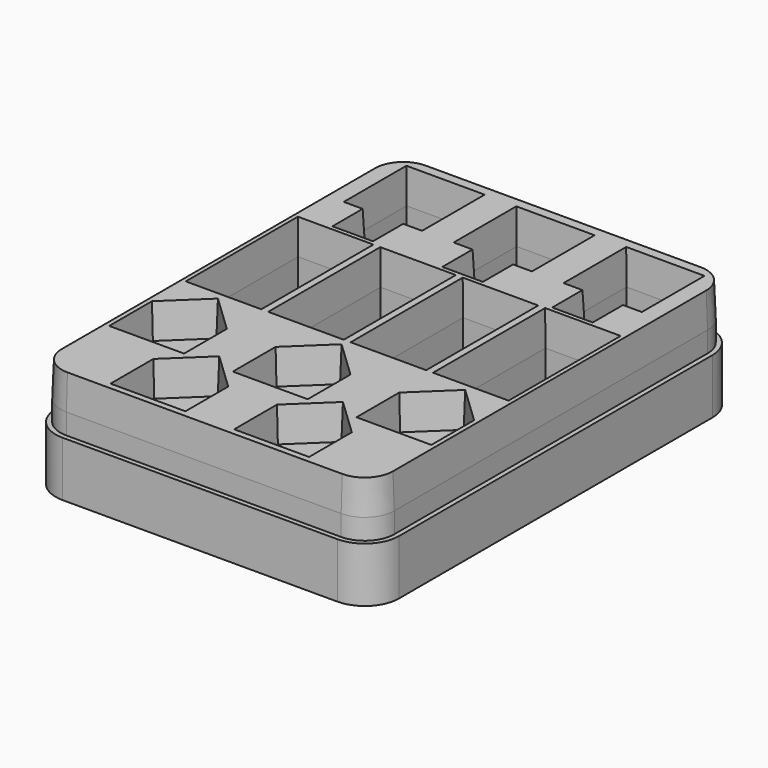
from build123d import *

# Parameters (mm, degrees)
F1_DEPTH = 1
F0_W     = 10.6
F0_H     = 20
F2_DEPTH = 7
F3_DEPTH = 11
F4_DEPTH = 16
F5_DEPTH = 8
F6_SIZE2 = 4.99999
F6_SIZE  = 0.19999


# Not quite as in the source:
# - a fillet or chamfer is up to 0.001 mm smaller than in the source, because OpenCascade refuses the exact size


with BuildPart() as f1:
    # F0 (on Top) → F1 (new body)
    with BuildSketch(Plane.XY):
        Polygon((-18.75, 14.5), (-13.25, 14.5), (-13.25, 20), (-10.5, 20), (-10.5, 31), (-21.5, 31), (-21.5, 20), (-18.75, 20), align=None)
    extrude(amount=F1_DEPTH)



with BuildPart() as f1b:
    # F0 (on Top) → F1, piece 2 (new body)
    with BuildSketch(Plane.XY):
        Polygon((5.5, 31), (-5.5, 31), (-5.5, 20), (-2.75, 20), (-2.75, 14.5), (2.75, 14.5), (2.75, 20), (5.5, 20), align=None)
    extrude(amount=F1_DEPTH)


with BuildPart() as f1c:
    # F0 (on Top) → F1, piece 3 (new body)
    with BuildSketch(Plane.XY):
        Polygon((21.5, 31), (10.5, 31), (10.5, 20), (13.25, 20), (13.25, 14.5), (18.75, 14.5), (18.75, 20), (21.5, 20), align=None)
    extrude(amount=F1_DEPTH)


with BuildPart() as f2:
    # F0 (on Top) → F2 (new body)
    with BuildSketch(Plane.XY):
        with Locations((-18, 3.5)):
            Rectangle(F0_W, F0_H)
    extrude(amount=F2_DEPTH)


with BuildPart() as f2b:
    # F0 (on Top) → F2, piece 2 (new body)
    with BuildSketch(Plane.XY):
        with Locations((-6, 3.5)):
            Rectangle(F0_W, F0_H)
    extrude(amount=F2_DEPTH)


with BuildPart() as f2c:
    # F0 (on Top) → F2, piece 3 (new body)
    with BuildSketch(Plane.XY):
        with Locations((6, 3.5)):
            Rectangle(F0_W, F0_H)
    extrude(amount=F2_DEPTH)


with BuildPart() as f2d:
    # F0 (on Top) → F2, piece 4 (new body)
    with BuildSketch(Plane.XY):
        with Locations((18, 3.5)):
            Rectangle(F0_W, F0_H)
    extrude(amount=F2_DEPTH)


with BuildPart() as f3:
    # F0 (on Top) → F3 (new body)
    with BuildSketch(Plane.XY):
        Polygon((-18, -8), (-23.25, -13), (-23.25, -20.5), (-12.75, -20.5), (-12.75, -13), align=None)
    extrude(amount=F3_DEPTH)


with BuildPart() as f3b:
    # F0 (on Top) → F3, piece 2 (new body)
    with BuildSketch(Plane.XY):
        Polygon((-5.25, -13), (-5.25, -20.5), (5.25, -20.5), (5.25, -13), (0, -8), align=None)
    extrude(amount=F3_DEPTH)


with BuildPart() as f3c:
    # F0 (on Top) → F3, piece 3 (new body)
    with BuildSketch(Plane.XY):
        Polygon((12.75, -13), (12.75, -20.5), (23.25, -20.5), (23.25, -13), (18, -8), align=None)
    extrude(amount=F3_DEPTH)


with BuildPart() as f3d:
    # F0 (on Top) → F3, piece 4 (new body)
    with BuildSketch(Plane.XY):
        Polygon((14.25, -31.5), (14.25, -24), (9, -19), (3.75, -24), (3.75, -31.5), align=None)
    extrude(amount=F3_DEPTH)


with BuildPart() as f3e:
    # F0 (on Top) → F3, piece 5 (new body)
    with BuildSketch(Plane.XY):
        Polygon((-3.75, -31.5), (-3.75, -24), (-9, -19), (-14.25, -24), (-14.25, -31.5), align=None)
    extrude(amount=F3_DEPTH)


with BuildPart() as f1_1:
    add(f1.part)

    add(f1b.part)  # F4 merges F1b

    add(f1c.part)  # F4 merges F1c

    add(f2.part)  # F4 merges F2

    add(f2b.part)  # F4 merges F2b

    add(f2c.part)  # F4 merges F2c

    add(f2d.part)  # F4 merges F2d

    add(f3.part)  # F4 merges F3

    add(f3b.part)  # F4 merges F3b

    add(f3c.part)  # F4 merges F3c

    add(f3d.part)  # F4 merges F3d

    add(f3e.part)  # F4 merges F3e
    # F0 (on Top) → F4 (join)
    with BuildSketch(Plane.XY):
        with BuildLine():
            ThreePointArc((24.3, 28.5), (23.0405591591, 31.5405591591), (20, 32.8))
            Line((20, 32.8), (-20, 32.8))
            ThreePointArc((-20, 32.8), (-23.0405591591, 31.5405591591), (-24.3, 28.5))
            Line((-24.3, 28.5), (-24.3, -28.5))
            ThreePointArc((-24.3, -28.5), (-23.0405591591, -31.5405591591), (-20, -32.8))
            Line((-20, -32.8), (20, -32.8))
            ThreePointArc((20, -32.8), (23.0405591591, -31.5405591591), (24.3, -28.5))
            Line((24.3, -28.5), (24.3, 28.5))
        make_face()
        Polygon((-9, -19), (-3.75, -24), (-3.75, -31.5), (-14.25, -31.5), (-14.25, -24), align=None, mode=Mode.SUBTRACT)
        Polygon((-23.25, -20.5), (-23.25, -13), (-18, -8), (-12.75, -13), (-12.75, -20.5), align=None, mode=Mode.SUBTRACT)
        Polygon((9, -19), (14.25, -24), (14.25, -31.5), (3.75, -31.5), (3.75, -24), align=None, mode=Mode.SUBTRACT)
        Polygon((5.25, -20.5), (-5.25, -20.5), (-5.25, -13), (0, -8), (5.25, -13), align=None, mode=Mode.SUBTRACT)
        Polygon((23.25, -20.5), (12.75, -20.5), (12.75, -13), (18, -8), (23.25, -13), align=None, mode=Mode.SUBTRACT)
        with Locations((-18, 3.5)):
            Rectangle(F0_W, F0_H, mode=Mode.SUBTRACT)
        with Locations((-6, 3.5)):
            Rectangle(F0_W, F0_H, mode=Mode.SUBTRACT)
        Polygon((-13.25, 20), (-13.25, 14.5), (-18.75, 14.5), (-18.75, 20), (-21.5, 20), (-21.5, 31), (-10.5, 31), (-10.5, 20), align=None, mode=Mode.SUBTRACT)
        with Locations((6, 3.5)):
            Rectangle(F0_W, F0_H, mode=Mode.SUBTRACT)
        with Locations((18, 3.5)):
            Rectangle(F0_W, F0_H, mode=Mode.SUBTRACT)
        Polygon((-5.5, 20), (-5.5, 31), (5.5, 31), (5.5, 20), (2.75, 20), (2.75, 14.5), (-2.75, 14.5), (-2.75, 20), align=None, mode=Mode.SUBTRACT)
        Polygon((10.5, 20), (10.5, 31), (21.5, 31), (21.5, 20), (18.75, 20), (18.75, 14.5), (13.25, 14.5), (13.25, 20), align=None, mode=Mode.SUBTRACT)
    extrude(amount=F4_DEPTH)

    # F0 (on Top) → F5 (join)
    with BuildSketch(Plane.XY):
        with BuildLine():
            ThreePointArc((25, 28.5), (23.5355339059, 32.0355339059), (20, 33.5))
            Line((20, 33.5), (-20, 33.5))
            ThreePointArc((-20, 33.5), (-23.5355339059, 32.0355339059), (-25, 28.5))
            Line((-25, 28.5), (-25, -28.5))
            ThreePointArc((-25, -28.5), (-23.5355339059, -32.0355339059), (-20, -33.5))
            Line((-20, -33.5), (20, -33.5))
            ThreePointArc((20, -33.5), (23.5355339059, -32.0355339059), (25, -28.5))
            Line((25, -28.5), (25, 28.5))
        make_face()
        with BuildLine():
            Line((-20, 32.8), (20, 32.8))
            ThreePointArc((20, 32.8), (23.0405591591, 31.5405591591), (24.3, 28.5))
            Line((24.3, 28.5), (24.3, -28.5))
            ThreePointArc((24.3, -28.5), (23.0405591591, -31.5405591591), (20, -32.8))
            Line((20, -32.8), (-20, -32.8))
            ThreePointArc((-20, -32.8), (-23.0405591591, -31.5405591591), (-24.3, -28.5))
            Line((-24.3, -28.5), (-24.3, 28.5))
            ThreePointArc((-24.3, 28.5), (-23.0405591591, 31.5405591591), (-20, 32.8))
        make_face(mode=Mode.SUBTRACT)
    extrude(amount=F5_DEPTH)

    # F6 (size 0.2 and 5 in the source; OpenCascade refuses exactly that, so slightly less here)
    f6_edges = [f1_1.edges().sort_by_distance(p)[0] for p in [
        (23.040559, 31.540559, 16),
        (0, 32.8, 16),
        (-23.040559, 31.540559, 16),
        (-24.3, 0, 16),
        (-23.040559, -31.540559, 16),
        (0, -32.8, 16),
        (23.040559, -31.540559, 16),
        (24.3, 0, 16),
        (-6.375, -21.5, 16),
        (-3.75, -27.75, 16),
        (-9, -31.5, 16),
        (-14.25, -27.75, 16),
        (-11.625, -21.5, 16),
        (-23.25, -16.75, 16),
        (-20.625, -10.5, 16),
        (-15.375, -10.5, 16),
        (-12.75, -16.75, 16),
        (-18, -20.5, 16),
        (11.625, -21.5, 16),
        (14.25, -27.75, 16),
        (9, -31.5, 16),
        (3.75, -27.75, 16),
        (6.375, -21.5, 16),
        (0, -20.5, 16),
        (-5.25, -16.75, 16),
        (-2.625, -10.5, 16),
        (2.625, -10.5, 16),
        (5.25, -16.75, 16),
        (18, -20.5, 16),
        (12.75, -16.75, 16),
        (15.375, -10.5, 16),
        (20.625, -10.5, 16),
        (23.25, -16.75, 16),
        (-23.3, 3.5, 16),
        (-18, 13.5, 16),
        (-12.7, 3.5, 16),
        (-18, -6.5, 16),
        (-6, -6.5, 16),
        (-11.3, 3.5, 16),
        (-6, 13.5, 16),
        (-0.7, 3.5, 16),
        (-13.25, 17.25, 16),
        (-16, 14.5, 16),
        (-18.75, 17.25, 16),
        (-20.125, 20, 16),
        (-21.5, 25.5, 16),
        (-16, 31, 16),
        (-10.5, 25.5, 16),
        (-11.875, 20, 16),
        (6, -6.5, 16),
        (0.7, 3.5, 16),
        (6, 13.5, 16),
        (11.3, 3.5, 16),
        (18, -6.5, 16),
        (12.7, 3.5, 16),
        (18, 13.5, 16),
        (23.3, 3.5, 16),
        (-5.5, 25.5, 16),
        (0, 31, 16),
        (5.5, 25.5, 16),
        (4.125, 20, 16),
        (2.75, 17.25, 16),
        (0, 14.5, 16),
        (-2.75, 17.25, 16),
        (-4.125, 20, 16),
        (10.5, 25.5, 16),
        (16, 31, 16),
        (21.5, 25.5, 16),
        (20.125, 20, 16),
        (18.75, 17.25, 16),
        (16, 14.5, 16),
        (13.25, 17.25, 16),
        (11.875, 20, 16),
    ]]
    f6_side = f1_1.faces().sort_by_distance((0, -2.524734, 16))[0]
    chamfer(f6_edges, length=F6_SIZE, length2=F6_SIZE2, reference=f6_side)


solid = f1_1.part
